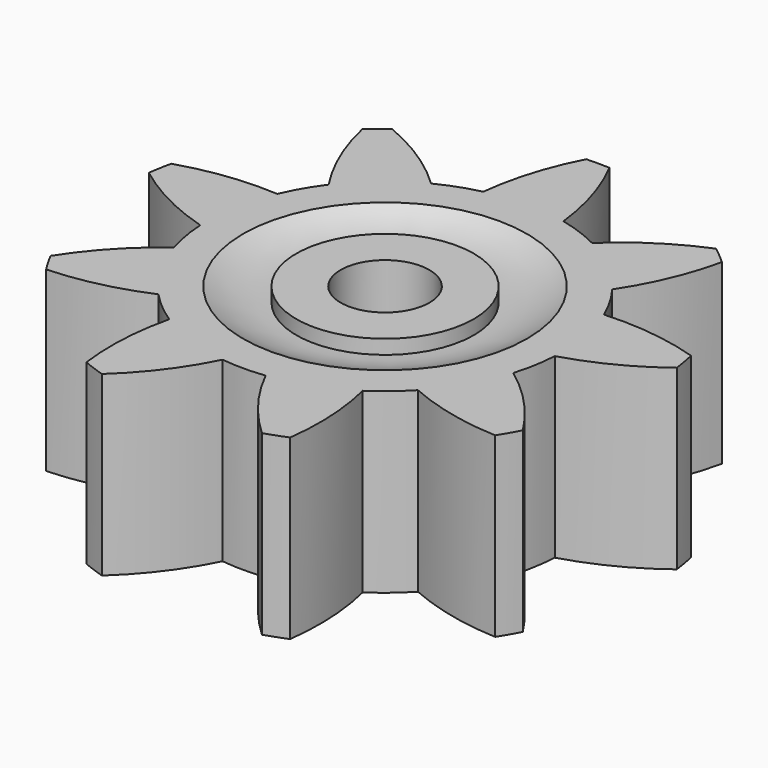
from build123d import *

# Parameters (mm, degrees)
F0_R     = 4.7625
F0_R_2   = 3.175
F0_R_3   = 1.5875
F1_DEPTH = 3.175
F2_R     = 5.08
F2_R_2   = 3.175
F3_DEPTH = 0.508
F4_R     = 5.08
F4_R_2   = 3.175
F5_DEPTH = 0.508


# Not quite as in the source:
# - a fillet or chamfer that OpenCascade refuses, or shapes differently, is made with other operations: its cross-section is extruded or revolved along the edge and cut away or added


with BuildPart() as f1:
    # F0 (on Top) → F1 (new body, symmetric)
    with BuildSketch(Plane.XY):
        with BuildLine():
            ThreePointArc((6.3411298165, -0.3355184801), (6.3477820668, -0.1678178556), (6.35, 0))
            ThreePointArc((6.35, 0), (6.222203729, 1.2675491134), (5.8439588173, 2.4840783686))
            ThreePointArc((5.8439588173, 2.4840783686), (5.499261314, 3.175), (5.0732543809, 3.8189776102))
            ThreePointArc((5.0732543809, 3.8189776102), (4.0817013215, 4.8643822138), (2.879997381, 5.6593387498))
            ThreePointArc((2.879997381, 5.6593387498), (2.1718279101, 5.967048142), (1.4315468375, 6.1865316335))
            ThreePointArc((1.4315468375, 6.1865316335), (0, 6.35), (-1.4315468375, 6.1865316335))
            ThreePointArc((-1.4315468375, 6.1865316335), (-2.1718279101, 5.967048142), (-2.879997381, 5.6593387498))
            ThreePointArc((-2.879997381, 5.6593387498), (-4.0817013215, 4.8643822138), (-5.0732543809, 3.8189776102))
            ThreePointArc((-5.0732543809, 3.8189776102), (-5.499261314, 3.175), (-5.8439588173, 2.4840783686))
            ThreePointArc((-5.8439588173, 2.4840783686), (-6.2535292316, 1.1026659282), (-6.3411298165, -0.3355184801))
            ThreePointArc((-6.3411298165, -0.3355184801), (-6.2535292316, -1.1026659282), (-6.0734669747, -1.8535098888))
            ThreePointArc((-6.0734669747, -1.8535098888), (-5.499261314, -3.175), (-4.6419201372, -4.3330217447))
            ThreePointArc((-4.6419201372, -4.3330217447), (-4.0817013215, -4.8643822138), (-3.4611324355, -5.3238202697))
            ThreePointArc((-3.4611324355, -5.3238202697), (-2.1718279101, -5.967048142), (-0.7707044365, -6.3030559788))
            ThreePointArc((-0.7707044365, -6.3030559788), (0, -6.35), (0.7707044365, -6.3030559788))
            ThreePointArc((0.7707044365, -6.3030559788), (2.1718279101, -5.967048142), (3.4611324355, -5.3238202697))
            ThreePointArc((3.4611324355, -5.3238202697), (4.0817013215, -4.8643822138), (4.6419201372, -4.3330217447))
            ThreePointArc((4.6419201372, -4.3330217447), (5.499261314, -3.175), (6.0734669747, -1.8535098888))
            ThreePointArc((6.0734669747, -1.8535098888), (6.2535292316, -1.1026659282), (6.3411298165, -0.3355184801))
        make_face()
        Circle(F0_R, mode=Mode.SUBTRACT)
        Circle(F0_R)
        Circle(F0_R_2, mode=Mode.SUBTRACT)
        Circle(F0_R_2)
        Circle(F0_R_3, mode=Mode.SUBTRACT)
        with BuildLine():
            ThreePointArc((5.8439588173, 2.4840783686), (6.222203729, 1.2675491134), (6.35, 0))
            ThreePointArc((6.35, 0), (6.3477820668, -0.1678178556), (6.3411298165, -0.3355184801))
            ThreePointArc((6.3411298165, -0.3355184801), (7.9650557648, 0.3109444224), (9.4435123046, 1.2432619809))
            ThreePointArc((9.4435123046, 1.2432619809), (9.3802938474, 1.6539988923), (9.2992194678, 2.0615873228))
            ThreePointArc((9.2992194678, 2.0615873228), (7.5910533822, 2.4320173351), (5.8439588173, 2.4840783686))
        make_face()
        with BuildLine():
            ThreePointArc((2.879997381, 5.6593387498), (4.0817013215, 4.8643822138), (5.0732543809, 3.8189776102))
            ThreePointArc((5.0732543809, 3.8189776102), (5.9017154857, 5.358036403), (6.4349967275, 7.0225666331))
            ThreePointArc((6.4349967275, 7.0225666331), (6.1225519823, 7.2965733207), (5.7984526113, 7.5566905663))
            ThreePointArc((5.7984526113, 7.5566905663), (4.2518136514, 6.7424684237), (2.879997381, 5.6593387498))
        make_face()
        with BuildLine():
            ThreePointArc((8.448778186, -4.3981555411), (7.3783548704, -3.0164016935), (6.0734669747, -1.8535098888))
            ThreePointArc((6.0734669747, -1.8535098888), (5.499261314, -3.175), (4.6419201372, -4.3330217447))
            ThreePointArc((4.6419201372, -4.3330217447), (6.3014579298, -4.8816419092), (8.0333035214, -5.1177787695))
            ThreePointArc((8.0333035214, -5.1177787695), (8.248891971, -4.7625), (8.448778186, -4.3981555411))
        make_face()
        with BuildLine():
            ThreePointArc((-1.4315468375, 6.1865316335), (0, 6.35), (1.4315468375, 6.1865316335))
            ThreePointArc((1.4315468375, 6.1865316335), (1.0768969406, 7.8980436026), (0.4154746647, 9.5159343106))
            ThreePointArc((0.4154746647, 9.5159343106), (0, 9.525), (-0.4154746647, 9.5159343106))
            ThreePointArc((-0.4154746647, 9.5159343106), (-1.0768969406, 7.8980436026), (-1.4315468375, 6.1865316335))
        make_face()
        with BuildLine():
            ThreePointArc((3.6450596933, -8.7999525472), (3.7132421134, -7.0534128461), (3.4611324355, -5.3238202697))
            ThreePointArc((3.4611324355, -5.3238202697), (2.1718279101, -5.967048142), (0.7707044365, -6.3030559788))
            ThreePointArc((0.7707044365, -6.3030559788), (1.6893378965, -7.790053738), (2.8642227403, -9.0841539559))
            ThreePointArc((2.8642227403, -9.0841539559), (3.2577418652, -8.950572213), (3.6450596933, -8.7999525472))
        make_face()
        with BuildLine():
            ThreePointArc((-5.0732543809, 3.8189776102), (-4.0817013215, 4.8643822138), (-2.879997381, 5.6593387498))
            ThreePointArc((-2.879997381, 5.6593387498), (-4.2518136514, 6.7424684237), (-5.7984526113, 7.5566905663))
            ThreePointArc((-5.7984526113, 7.5566905663), (-6.1225519823, 7.2965733207), (-6.4349967275, 7.0225666331))
            ThreePointArc((-6.4349967275, 7.0225666331), (-5.9017154857, 5.358036403), (-5.0732543809, 3.8189776102))
        make_face()
        with BuildLine():
            ThreePointArc((-2.8642227403, -9.0841539559), (-1.6893378965, -7.790053738), (-0.7707044365, -6.3030559788))
            ThreePointArc((-0.7707044365, -6.3030559788), (-2.1718279101, -5.967048142), (-3.4611324355, -5.3238202697))
            ThreePointArc((-3.4611324355, -5.3238202697), (-3.7132421134, -7.0534128461), (-3.6450596933, -8.7999525472))
            ThreePointArc((-3.6450596933, -8.7999525472), (-3.2577418652, -8.950572213), (-2.8642227403, -9.0841539559))
        make_face()
        with BuildLine():
            ThreePointArc((-6.3411298165, -0.3355184801), (-6.2535292316, 1.1026659282), (-5.8439588173, 2.4840783686))
            ThreePointArc((-5.8439588173, 2.4840783686), (-7.5910533822, 2.4320173351), (-9.2992194678, 2.0615873228))
            ThreePointArc((-9.2992194678, 2.0615873228), (-9.3802938474, 1.6539988923), (-9.4435123046, 1.2432619809))
            ThreePointArc((-9.4435123046, 1.2432619809), (-7.9650557648, 0.3109444224), (-6.3411298165, -0.3355184801))
        make_face()
        with BuildLine():
            ThreePointArc((-8.0333035214, -5.1177787695), (-6.3014579298, -4.8816419092), (-4.6419201372, -4.3330217447))
            ThreePointArc((-4.6419201372, -4.3330217447), (-5.499261314, -3.175), (-6.0734669747, -1.8535098888))
            ThreePointArc((-6.0734669747, -1.8535098888), (-7.3783548704, -3.0164016935), (-8.448778186, -4.3981555411))
            ThreePointArc((-8.448778186, -4.3981555411), (-8.248891971, -4.7625), (-8.0333035214, -5.1177787695))
        make_face()
    extrude(amount=F1_DEPTH, both=True)

    # F2 (on face) → F3 (cut)
    with BuildSketch(Plane(origin=(0, 0, -3.175), x_dir=(1, 0, 0), z_dir=(0, 0, -1))):
        Circle(F2_R)
        Circle(F2_R_2, mode=Mode.SUBTRACT)
    extrude(amount=-F3_DEPTH, mode=Mode.SUBTRACT)

    # F4 (on face) → F5 (cut)
    with BuildSketch(Plane.XY.offset(3.175)):
        Circle(F4_R)
        Circle(F4_R_2, mode=Mode.SUBTRACT)
    extrude(amount=-F5_DEPTH, mode=Mode.SUBTRACT)

    # F6: fillet of radius 3.81 on 2 edges, made by hand

    # F6_s1 → F6_t2 (revolve)
    with BuildSketch(Plane.XZ):
        with BuildLine():
            ThreePointArc((5.08, 3.175), (4.1629758175, 2.7961903065), (3.1792380475, 2.667))
            Line((3.1792380475, 2.667), (5.08, 2.667))
            Line((5.08, 2.667), (5.08, 3.175))
        make_face()
    revolve(axis=Axis((0, 0, 2.667), (0, 0, 1)))

    # F6_s3 → F6_t4 (revolve)
    with BuildSketch(Plane.XZ):
        with BuildLine():
            ThreePointArc((5.08, -3.175), (4.1629758175, -2.7961903065), (3.1792380475, -2.667))
            Line((3.1792380475, -2.667), (5.08, -2.667))
            Line((5.08, -2.667), (5.08, -3.175))
        make_face()
    revolve(axis=Axis((0, 0, -2.667), (0, 0, -1)))


solid = f1.part
